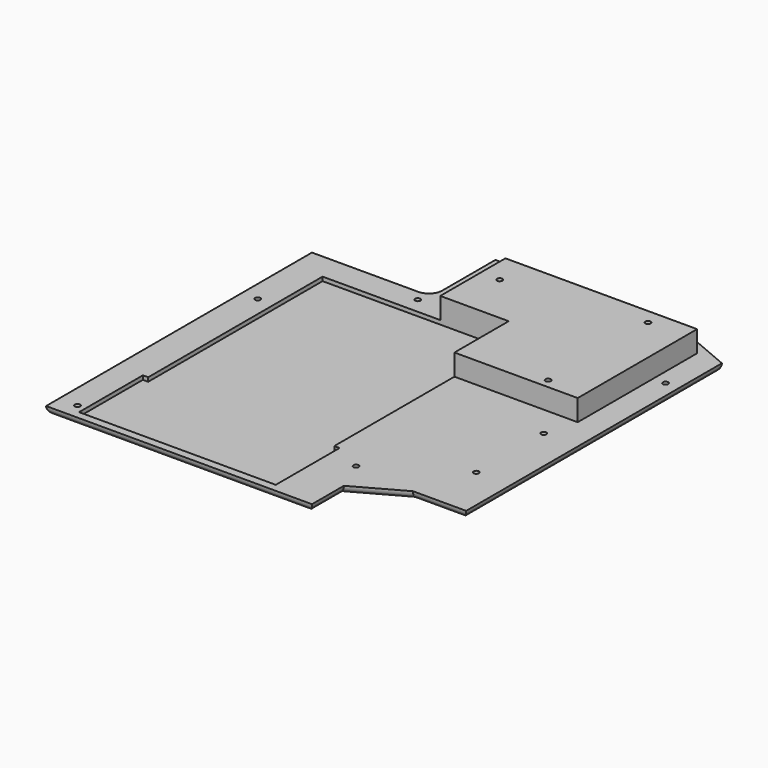
from build123d import *

# Parameters (mm, degrees)
F0_W      = 45
F0_H      = 110
F0_H_2    = 15
F0_W_2    = 20
F0_H_3    = 100
F0_W_3    = 55
F1_DEPTH  = 3
F2_R      = 5
F3_R      = 2.99999
F5_D      = 2
F6_W      = 70
F6_H      = 82
F7_DEPTH  = 1.5
F8_W      = 46.3650951658
F8_H      = 25.5117665604
F9_DEPTH  = 8
F11_D     = 2
F11_DEPTH = 6
F11_TIP   = 0.600860619


# Not quite as in the source:
# - a fillet or chamfer is up to 0.001 mm smaller than in the source, because OpenCascade refuses the exact size


with BuildPart() as f1:
    # F0 (on Top) → F1 (new body)
    with BuildSketch(Plane.XY):
        with Locations((-49.1538274859, -4.7530609369)):
            Rectangle(F0_W, F0_H)
        Polygon((43.3461725141, 50.2469390631), (-26.6538274859, 50.2469390631), (-26.6538274859, -59.7530609369), (28.3461725141, -59.7530609369), (46.3587938504, -49.7530609369), (46.3587938504, 50.2469390631), align=None)
        with Locations((-49.1538274859, -67.2530609369)):
            Rectangle(F0_W, F0_H_2)
        with Locations((56.3587938504, 0.2469390631)):
            Rectangle(F0_W_2, F0_H_3)
        with Locations((0.8461725141, -67.2530609369)):
            Rectangle(F0_W_3, F0_H_2)
        Polygon((-26.6538274859, 80.2469390631), (-26.6538274859, 50.2469390631), (43.3461725141, 50.2469390631), (43.3461725141, 70.4786608508), (43.3461725141, 80.2469390631), align=None)
        Polygon((43.3461725141, 70.4786608508), (43.3461725141, 50.2469390631), (46.3587938504, 50.2469390631), (66.3587938504, 50.2469390631), (66.3587938504, 70.4786608508), align=None)
        Polygon((43.3461725141, 80.2469390631), (43.3461725141, 70.4786608508), (66.3587938504, 70.4786608508), align=None)
    extrude(amount=F1_DEPTH)

    # F2
    f2_edges = [f1.edges().sort_by_distance(p)[0] for p in [
        (-26.653827, 50.246939, 1.5),
    ]]
    fillet(f2_edges, radius=F2_R)

    # F3 (radius 3 in the source; OpenCascade refuses exactly that, so slightly less here)
    f3_edges = [f1.edges().sort_by_distance(p)[0] for p in [
        (-26.653827, 67.746939, 0),
        (-28.118294, 51.711405, 0),
        (8.346173, 80.246939, 0),
        (-51.653827, 50.246939, 0),
        (54.852483, 75.3628, 0),
        (-71.653827, -12.253061, 0),
        (66.358794, 10.3628, 0),
        (-21.653827, -74.753061, 0),
        (56.358794, -49.753061, 0),
        (28.346173, -67.253061, 0),
        (37.352483, -54.753061, 0),
    ]]
    fillet(f3_edges, radius=F3_R)

    # F5 (through all)
    with Locations(Plane.XY.offset(3)):
        with Locations((-65.6538274859, 17.2469390631), (-64.6538274859, -68.7530609369), (23.3461725141, -47.7530609369), (53.3587938504, -28.7530609369), (53.3587938504, 2.9659790631), (61.3461725141, 50.2469390631), (33.3461725141, 74.2469390631), (-28.6538274859, 46.2469390631)):
            Hole(F5_D / 2)

    # F6 (on face) → F7 (cut)
    with BuildSketch(Plane.XY.offset(3)):
        with Locations((-24.6538274859, -0.7530609369)):
            Rectangle(F6_W, F6_H)
        Polygon((-61.6538274859, -41.7530609369), (-61.6538274859, -71.7530609369), (12.3461725141, -71.7530609369), (12.3461725141, -41.7530609369), (10.3461725141, -41.7530609369), (-59.6538274859, -41.7530609369), align=None)
    extrude(amount=-F7_DEPTH, mode=Mode.SUBTRACT)

    # F8 (on face) → F9 (join)
    with BuildSketch(Plane.XY.offset(3)):
        Polygon((-15.3889879584, 70.8764791489), (-15.3889879584, 40.2469390631), (10.3461725141, 40.2469390631), (56.7112676799, 40.2469390631), (56.7112676799, 70.8764791489), align=None)
        with Locations((33.528720097, 27.4910557829)):
            Rectangle(F8_W, F8_H)
    extrude(amount=F9_DEPTH)

    # F11
    with Locations(Plane.XY.offset(11)):
        with Locations((-8.1770029031, 59.1886730194), (42.8229970969, 65.1886730194), (42.8229970969, 18.1886730194)):
            Hole(F11_D / 2, depth=F11_DEPTH)
            with Locations((0, 0, -(F11_DEPTH + F11_TIP / 2))):  # 118° drill point
                Cone(0, F11_D / 2, F11_TIP, mode=Mode.SUBTRACT)


solid = f1.part
